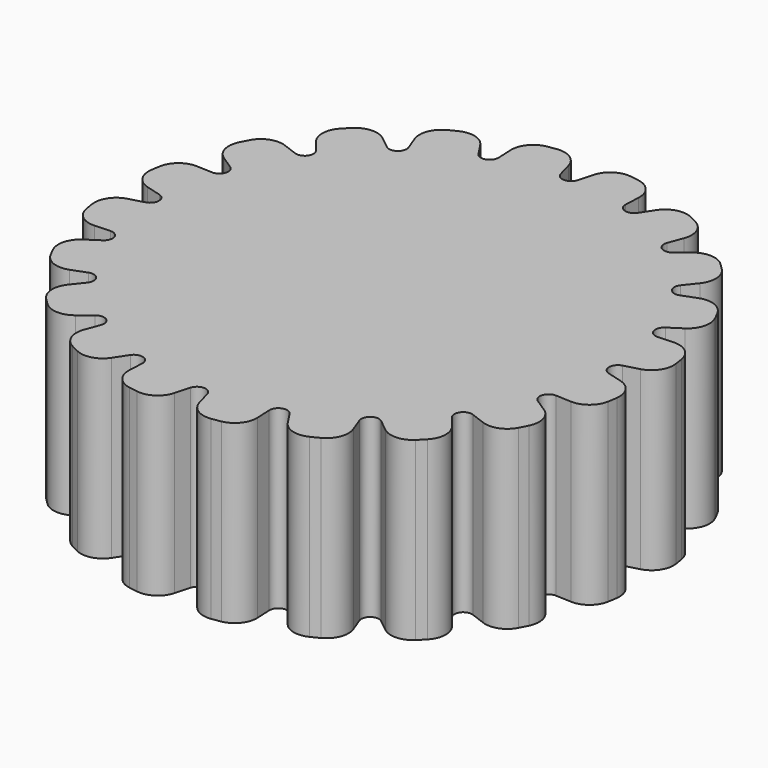
from build123d import *

# Parameters (mm, degrees)
F0_R            = 76.3894607231
F1_DEPTH        = 25.4
F2_DEPTH        = 25.4
F4_DEPTH        = 50.8
F4_COPIES_COUNT = 20
F5_R            = 6.35
F6_R            = 2.54


# Not quite as in the source:
# - a pattern or mirror of a feature is missing from the dataset's text; its kind, count and spacing are read off the source's solid


with BuildPart() as f1:
    # F0 (on Top) → F1 (new body)
    with BuildSketch(Plane.XY):
        Circle(F0_R)
    extrude(amount=F1_DEPTH)

    # F2 (add): a face of the model
    f2_faces = [f1.faces().sort_by_distance(p)[0] for p in [
        (0, 0, 25.4),
    ]]
    extrude(f2_faces, amount=F2_DEPTH)

    # F3 (on face) → F4 (cut)
    with BuildSketch(Plane.XY.offset(50.8)):
        with BuildLine():
            ThreePointArc((5.0502526328, 76.2223370011), (-0.0057278173, 76.3894605084), (-5.0616831482, 76.2215787902))
            Line((-5.0616831482, 76.2215787902), (0, 57.8660437425))
            Line((0, 57.8660437425), (5.0502526328, 76.2223370011))
        make_face()
    f4 = extrude(amount=-F4_DEPTH, mode=Mode.SUBTRACT)

    # F4_copies: F4 ×20 about axis
    f4_copies_axis = Axis((0, 0, 0), (0, 0, 1))
    for i in range(1, F4_COPIES_COUNT):
        add(f4.rotate(f4_copies_axis, i * 360 / F4_COPIES_COUNT), mode=Mode.SUBTRACT)

    # F5
    f5_edges = [f1.edges().sort_by_distance(p)[0] for p in [
        (-5.061683, 76.221579, 25.4),
        (5.050253, 76.222337, 25.4),
        (-18.750922, 74.052364, 25.4),
        (18.739816, 74.055175, 25.4),
        (28.357073, 70.931136, 25.4),
        (40.706932, 64.639735, 25.4),
        (48.888106, 58.696702, 25.4),
        (58.68937, 48.896908, 25.4),
        (64.63363, 40.716625, 25.4),
        (70.926883, 28.36771, 25.4),
        (74.052364, 18.750922, 25.4),
        (76.221579, 5.061683, 25.4),
        (76.222337, -5.050253, 25.4),
        (74.055175, -18.739816, 25.4),
        (70.931136, -28.357073, 25.4),
        (64.639735, -40.706932, 25.4),
        (58.696702, -48.888106, 25.4),
        (48.896908, -58.68937, 25.4),
        (40.716625, -64.63363, 25.4),
        (28.36771, -70.926883, 25.4),
        (18.750922, -74.052364, 25.4),
        (5.061683, -76.221579, 25.4),
        (-5.050253, -76.222337, 25.4),
        (-18.739816, -74.055175, 25.4),
        (-28.357073, -70.931136, 25.4),
        (-40.706932, -64.639735, 25.4),
        (-48.888106, -58.696702, 25.4),
        (-58.68937, -48.896908, 25.4),
        (-64.63363, -40.716625, 25.4),
        (-70.926883, -28.36771, 25.4),
        (-74.052364, -18.750922, 25.4),
        (-76.221579, -5.061683, 25.4),
        (-76.222337, 5.050253, 25.4),
        (-74.055175, 18.739816, 25.4),
        (-70.931136, 28.357073, 25.4),
        (-64.639735, 40.706932, 25.4),
        (-58.696702, 48.888106, 25.4),
        (-48.896908, 58.68937, 25.4),
        (-40.716625, 64.63363, 25.4),
        (-28.36771, 70.926883, 25.4),
    ]]
    fillet(f5_edges, radius=F5_R)

    # F6
    f6_edges = [f1.edges().sort_by_distance(p)[0] for p in [
        (0, 57.866044, 25.4),
        (-17.881591, 55.033878, 25.4),
        (17.881591, 55.033878, 25.4),
        (-34.012807, 46.814613, 25.4),
        (34.012807, 46.814613, 25.4),
        (-46.814613, 34.012807, 25.4),
        (46.814613, 34.012807, 25.4),
        (-55.033878, 17.881591, 25.4),
        (55.033878, 17.881591, 25.4),
        (-57.866044, 0, 25.4),
        (57.866044, 0, 25.4),
        (-55.033878, -17.881591, 25.4),
        (55.033878, -17.881591, 25.4),
        (-46.814613, -34.012807, 25.4),
        (46.814613, -34.012807, 25.4),
        (-34.012807, -46.814613, 25.4),
        (34.012807, -46.814613, 25.4),
        (-17.881591, -55.033878, 25.4),
        (17.881591, -55.033878, 25.4),
        (0, -57.866044, 25.4),
    ]]
    fillet(f6_edges, radius=F6_R)


solid = f1.part
